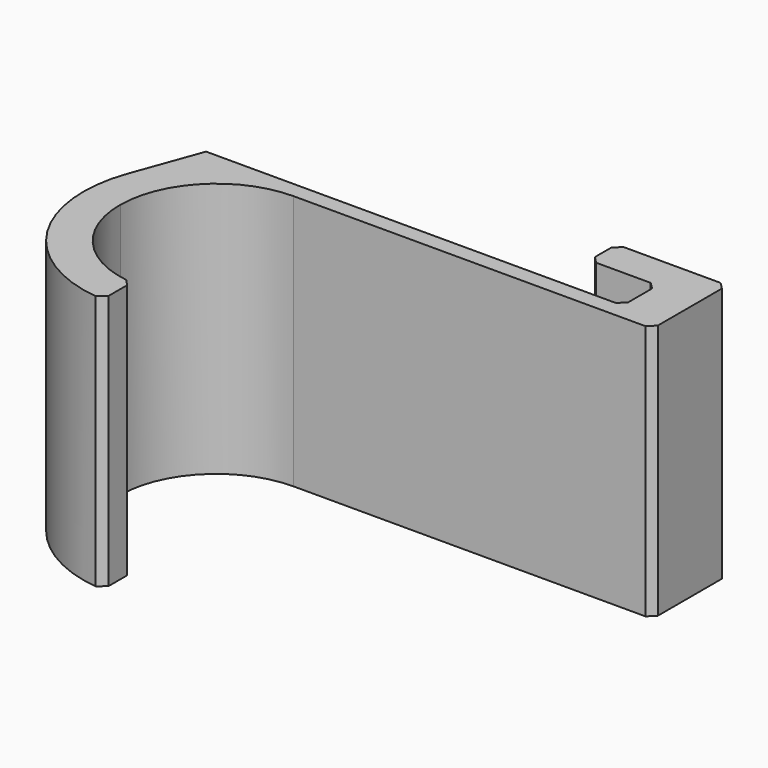
from build123d import *

# Parameters (mm, degrees)
F1_DEPTH    = 30
F2_T1_DEPTH = 30
F2_T3_DEPTH = 34.1146927807
F2_T5_DEPTH = 34.5796675935
F2_T7_DEPTH = 33.7107882322


# Not quite as in the source:
# - a fillet or chamfer that OpenCascade refuses, or shapes differently, is made with other operations: its cross-section is extruded or revolved along the edge and cut away or added


with BuildPart() as f1:
    # F0 (on Top) → F1 (new body)
    with BuildSketch(Plane.XY):
        with BuildLine():
            Line((0, 4), (0, 0))
            Line((0, 0), (8, 0))
            Line((8, 0), (8, -5.11398))
            Line((8, -5.11398), (0, -5.11398))
            Line((0, -5.11398), (-30, -5.11398))
            Line((-30, -5.11398), (-40.9191332404, -5.11398))
            Line((-40.9191332404, -5.11398), (-43.7934957599, -13.012435493))
            ThreePointArc((-43.7934957599, -13.012435493), (-44.486999636, -15.5813060668), (-44.7341086379, -18.230641982))
            ThreePointArc((-44.7341086379, -18.230641982), (-40.5087550106, -29.0303309912), (-30, -33.9347131233))
            Line((-30, -33.9347131233), (-30, -29.6540509196))
            ThreePointArc((-30, -29.6540509196), (-37.4863926883, -26.0077839606), (-40.4625312712, -18.230641982))
            ThreePointArc((-40.4625312712, -18.230641982), (-37.1000637613, -10.2912492126), (-29.125629618, -7.0127517826))
            Line((-29.125629618, -7.0127517826), (0, -7.0127517826))
            Line((0, -7.0127517826), (13, -7.0127517826))
            Line((13, -7.0127517826), (13, 4))
            Line((13, 4), (0, 4))
        make_face()
    extrude(amount=F1_DEPTH)

    # F2: chamfer of 0.8 on 8 edges, made by hand

    # F2_s2 → F2_t1 (join)
    with BuildSketch(Plane.XY):
        Polygon((8, -0.8), (7.2, 0), (8, 0), align=None)
        Polygon((7.2, -5.11398), (8, -4.31398), (8, -5.11398), align=None)
    extrude(amount=F2_T1_DEPTH)

    # F2_s4 → F2_t3 (cut)
    with BuildSketch(Plane.XY.offset(-2.0573463904)):
        Polygon((0, 0.8), (0.8, 0), (0, 0), align=None)
        Polygon((0.8, 4), (0, 3.2), (0, 4), align=None)
        Polygon((12.2, -7.0127517826), (13, -6.2127517826), (13, -7.0127517826), align=None)
        Polygon((13, 3.2), (12.2, 4), (13, 4), align=None)
    extrude(amount=F2_T3_DEPTH, mode=Mode.SUBTRACT)

    # F2_s6 → F2_t5 (cut)
    with BuildSketch(Plane.XY.offset(-2.2898337967)):
        with BuildLine():
            Line((-30.8904518842, -33.859131698), (-30, -33.0642616101))
            Line((-30, -33.0642616101), (-30, -33.9347131233))
            ThreePointArc((-30, -33.9347131233), (-30.4567158355, -33.9023630924), (-30.8904518842, -33.859131698))
        make_face()
    extrude(amount=F2_T5_DEPTH, mode=Mode.SUBTRACT)

    # F2_s8 → F2_t7 (cut)
    with BuildSketch(Plane.XY.offset(-1.8553941161)):
        with BuildLine():
            Line((-30, -30.3717734146), (-30.6896401509, -29.5794220382))
            ThreePointArc((-30.6896401509, -29.5794220382), (-30.3570806998, -29.6207408817), (-30, -29.6540509196))
            Line((-30, -29.6540509196), (-30, -30.3717734146))
        make_face()
    extrude(amount=F2_T7_DEPTH, mode=Mode.SUBTRACT)


solid = f1.part
